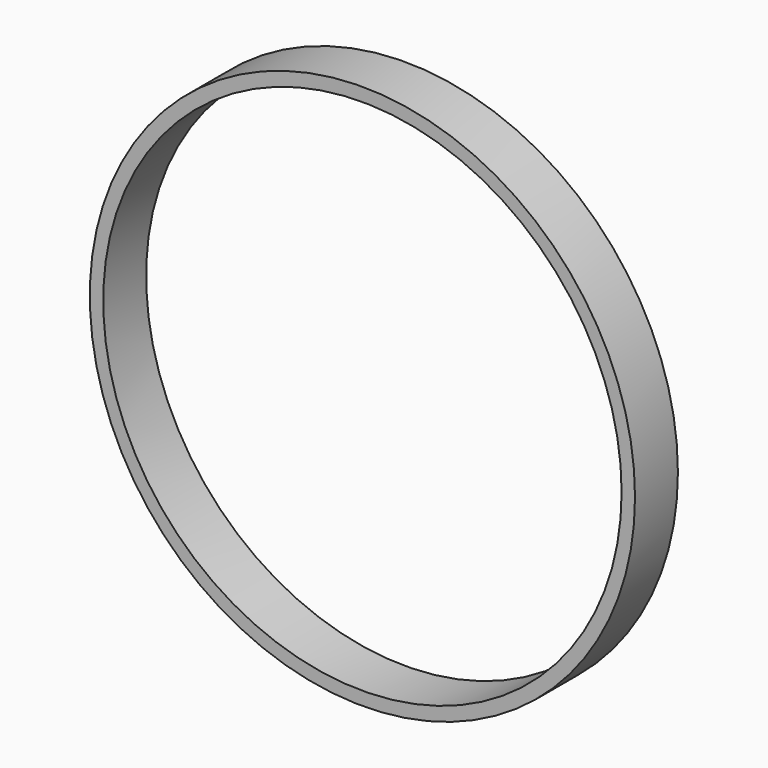
from build123d import *

# Parameters (mm, degrees)
F0_R     = 15.25
F0_R_2   = 14.5
F2_DEPTH = 3


# Not quite as in the source:
# - the program builds the solid bodies; features that only make, move or delete a surface that nothing else refers to are left out


with BuildPart() as f2:
    # F0 (on Front) → F2 (new body)
    with BuildSketch(Plane.XZ):
        Circle(F0_R)
        Circle(F0_R_2, mode=Mode.SUBTRACT)
    extrude(amount=F2_DEPTH)


solid = f2.part
